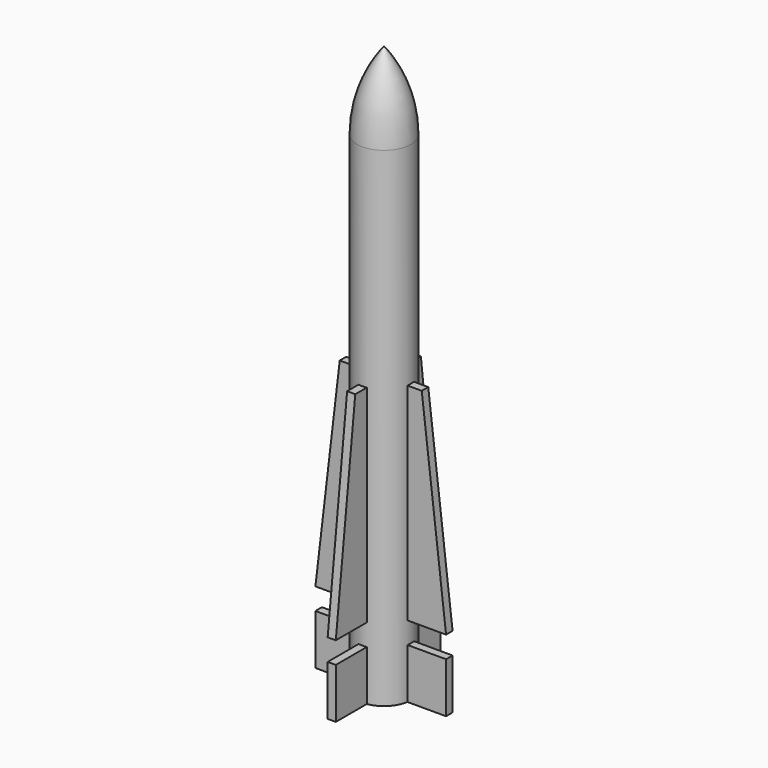
from build123d import *

# Parameters (mm, degrees)
F3_DEPTH = 0.2
F4_COUNT = 4


# Not quite as in the source:
# - a feature names something its author has since deleted; it is built from what else it names


with BuildPart() as f1:
    # F0 (on Front) → F1 (revolve)
    with BuildSketch(Plane.XZ):
        with BuildLine():
            Line((0, 27.8472222222), (0, 0))
            Line((0, 0), (1.3229166667, 0))
            Line((1.3229166667, 0), (1.3229166667, 24.0277777778))
            ThreePointArc((1.3229166667, 24.0277777778), (0.9828221086, 26.0488087258), (0, 27.8472222222))
        make_face()
    revolve(axis=Axis((0, 0, 13.9236111111), (0, 0, 1)))

    # F2 (on Front) → F3 (join, symmetric)
    with BuildSketch(Plane.XZ):
        Polygon((0, 13.6805555556), (0, 0), (1.3229166667, 0), (3.2083333333, 0), (3.2083333333, 2.4652777778), (0.4, 2.4652777778), (0.4, 3.5277777778), (3.2083333333, 3.5277777778), (2.0138888889, 13.6805555556), align=None)
    extrude(amount=F3_DEPTH, both=True)

    # F4: F1 ×4 about axis
    f4_axis = Axis((0, 0, 0), (0, 0, 1))


with BuildPart() as f1_1:
    add(f1.part)
    for i in range(1, F4_COUNT):
        add(f1.part.rotate(f4_axis, i * 360 / F4_COUNT))


solid = f1_1.part
